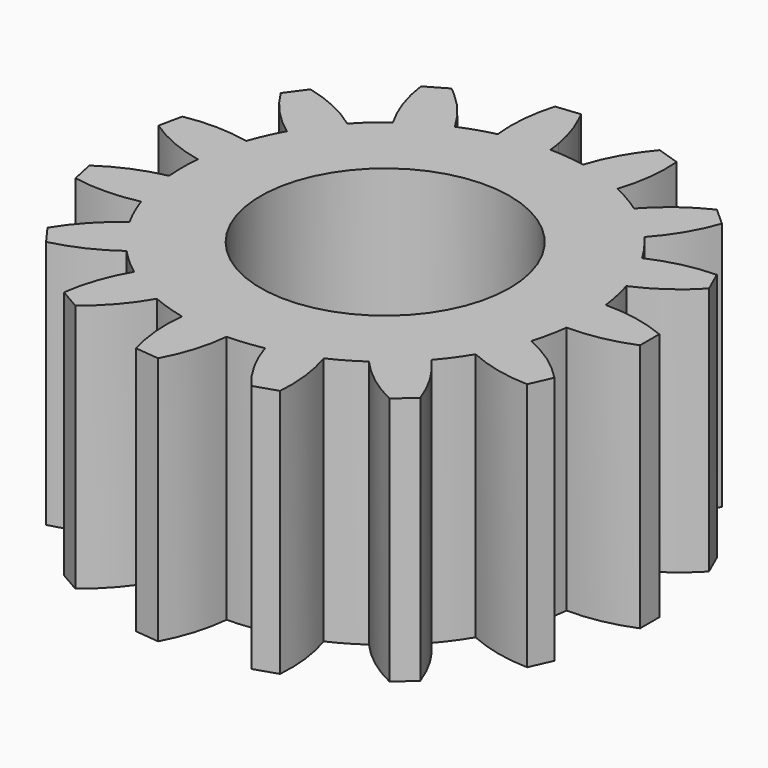
from build123d import *

# Parameters (mm, degrees)
F1_R     = 2
F2_DEPTH = 4


# Not quite as in the source:
# - a feature names something its author has since deleted; it is built from what else it names


with BuildPart() as f2:
    # F1 (on Top) → F2 (new body)
    with BuildSketch(Plane.XY):
        with BuildLine():
            ThreePointArc((-0.009331824, 3.2499866026), (0.0217852654, 3.2499269841), (0.0529003577, 3.249569441))
            ThreePointArc((0.0529003577, 3.249569441), (0.0415378352, 3.3466273722), (0.0265550076, 3.4431927066))
            ThreePointArc((0.0265550076, 3.4431927066), (0.0136878461, 3.345646772), (-0.009331824, 3.2499866026))
        make_face()
        with BuildLine():
            ThreePointArc((-0.7273678349, 3.1675599494), (-0.3706482634, 3.2287954201), (-0.009331824, 3.2499866026))
            ThreePointArc((-0.009331824, 3.2499866026), (0.0136878461, 3.345646772), (0.0265550076, 3.4431927066))
            ThreePointArc((0.0265550076, 3.4431927066), (-0.0579521884, 3.7877136915), (-0.1883330995, 4.1176182129))
            ThreePointArc((-0.1883330995, 4.1176182129), (-0.2452042442, 4.1798359688), (-0.3074340323, 4.2366939473))
            Line((-0.3074340323, 4.2366939473), (-0.6356215278, 4.2022000516))
            ThreePointArc((-0.6356215278, 4.2022000516), (-0.733410077, 3.6894835779), (-0.7273678349, 3.1675599494))
        make_face()
        with BuildLine():
            ThreePointArc((-0.3074340323, 4.2366939473), (-0.2452042442, 4.1798359688), (-0.1883330995, 4.1176182129))
            ThreePointArc((-0.1883330995, 4.1176182129), (-0.219306435, 4.1804982316), (-0.2519548455, 4.2425250448))
            Line((-0.2519548455, 4.2425250448), (-0.3074340323, 4.2366939473))
        make_face()
        with BuildLine():
            ThreePointArc((3.2262383665, -0.392283064), (3.2440541527, -0.1965010289), (3.25, 0))
            ThreePointArc((3.25, 0), (3.2440541527, 0.1965010289), (3.2262383665, 0.392283064))
            ThreePointArc((3.2262383665, 0.392283064), (3.1789797024, 0.6757129952), (3.1068713016, 0.9538609518))
            ThreePointArc((3.1068713016, 0.9538609518), (2.9690227373, 1.32189409), (2.7877595085, 1.6705977742))
            ThreePointArc((2.7877595085, 1.6705977742), (2.6293052317, 1.91030207), (2.4502979636, 2.1350737434))
            ThreePointArc((2.4502979636, 2.1350737434), (2.1746744707, 2.4152206828), (1.8672517054, 2.6600509523))
            ThreePointArc((1.8672517054, 2.6600509523), (1.625, 2.8145825623), (1.3700458474, 2.9471128883))
            ThreePointArc((1.3700458474, 2.9471128883), (1.0043052317, 3.090933678), (0.623879119, 3.189557155))
            ThreePointArc((0.623879119, 3.189557155), (0.3397175056, 3.2321961599), (0.0529003577, 3.249569441))
            ThreePointArc((0.0529003577, 3.249569441), (0.0217852654, 3.2499269841), (-0.009331824, 3.2499866026))
            ThreePointArc((-0.009331824, 3.2499866026), (-0.673671928, 2.6091227037), (-1.565226307, 2.8482567665))
            ThreePointArc((-1.565226307, 2.8482567665), (-1.7634860259, 2.7299481747), (-1.9528462821, 2.5978628521))
            ThreePointArc((-1.9528462821, 2.5978628521), (-2.1746744707, 2.4152206828), (-2.3795034667, 2.2136989976))
            ThreePointArc((-2.3795034667, 2.2136989976), (-2.6293052317, 1.91030207), (-2.8406598662, 1.5789716669))
            ThreePointArc((-2.8406598662, 1.5789716669), (-2.9690227373, 1.32189409), (-3.0741770825, 1.0544834116))
            ThreePointArc((-3.0741770825, 1.0544834116), (-3.1789797024, 0.6757129952), (-3.2372975527, 0.287061936))
            ThreePointArc((-3.2372975527, 0.287061936), (-3.25, 0), (-3.2372975527, -0.287061936))
            ThreePointArc((-3.2372975527, -0.287061936), (-3.1789797024, -0.6757129952), (-3.0741770825, -1.0544834116))
            ThreePointArc((-3.0741770825, -1.0544834116), (-2.9690227373, -1.32189409), (-2.8406598662, -1.5789716669))
            ThreePointArc((-2.8406598662, -1.5789716669), (-2.6293052317, -1.91030207), (-2.3795034667, -2.2136989976))
            ThreePointArc((-2.3795034667, -2.2136989976), (-2.1746744707, -2.4152206828), (-1.9528462821, -2.5978628521))
            ThreePointArc((-1.9528462821, -2.5978628521), (-1.625, -2.8145825623), (-1.2733920844, -2.9901459161))
            ThreePointArc((-1.2733920844, -2.9901459161), (-1.0043052317, -3.090933678), (-0.7273678349, -3.1675599494))
            ThreePointArc((-0.7273678349, -3.1675599494), (-0.3397175056, -3.2321961599), (0.0529003577, -3.249569441))
            ThreePointArc((0.0529003577, -3.249569441), (0.3397175056, -3.2321961599), (0.623879119, -3.189557155))
            ThreePointArc((0.623879119, -3.189557155), (1.0043052317, -3.090933678), (1.3700458474, -2.9471128883))
            ThreePointArc((1.3700458474, -2.9471128883), (1.625, -2.8145825623), (1.8672517054, -2.6600509523))
            ThreePointArc((1.8672517054, -2.6600509523), (2.1746744707, -2.4152206828), (2.4502979636, -2.1350737434))
            ThreePointArc((2.4502979636, -2.1350737434), (2.6293052317, -1.91030207), (2.7877595085, -1.6705977742))
            ThreePointArc((2.7877595085, -1.6705977742), (2.9690227373, -1.32189409), (3.1068713016, -0.9538609518))
            ThreePointArc((3.1068713016, -0.9538609518), (3.1789797024, -0.6757129952), (3.2262383665, -0.392283064))
        make_face()
        Circle(F1_R, mode=Mode.SUBTRACT)
        with BuildLine():
            ThreePointArc((-1.8325056355, 3.6726799025), (-1.7998502093, 3.2277290794), (-1.565226307, 2.8482567665))
            ThreePointArc((-1.565226307, 2.8482567665), (-1.4210811819, 2.9228459204), (-1.2733920844, 2.9901459161))
            ThreePointArc((-1.2733920844, 2.9901459161), (-1.5239397604, 3.3551763863), (-1.8325056355, 3.6726799025))
        make_face()
        with BuildLine():
            ThreePointArc((-1.9528462821, 2.5978628521), (-1.7634860259, 2.7299481747), (-1.565226307, 2.8482567665))
            ThreePointArc((-1.565226307, 2.8482567665), (-1.7998502093, 3.2277290794), (-1.8325056355, 3.6726799025))
            ThreePointArc((-1.8325056355, 3.6726799025), (-1.893368674, 3.7239080781), (-1.9557625995, 3.7732602156))
            Line((-1.9557625995, 3.7732602156), (-2.289857902, 3.5803702027))
            ThreePointArc((-2.289857902, 3.5803702027), (-2.1706516096, 3.0722062109), (-1.9528462821, 2.5978628521))
        make_face()
        with BuildLine():
            ThreePointArc((-2.8406598662, 1.5789716669), (-2.6293052317, 1.91030207), (-2.3795034667, 2.2136989976))
            ThreePointArc((-2.3795034667, 2.2136989976), (-2.8284814668, 2.4798935471), (-3.3214012325, 2.651564416))
            Line((-3.3214012325, 2.651564416), (-3.5481570423, 2.3394618192))
            ThreePointArc((-3.5481570423, 2.3394618192), (-3.2325677592, 1.9237164799), (-2.8406598662, 1.5789716669))
        make_face()
        with BuildLine():
            ThreePointArc((-3.2372975527, 0.287061936), (-3.1789797024, 0.6757129952), (-3.0741770825, 1.0544834116))
            ThreePointArc((-3.0741770825, 1.0544834116), (-3.5926099725, 1.1150484286), (-4.1127394185, 1.0713890403))
            Line((-4.1127394185, 1.0713890403), (-4.1929475959, 0.6940392338))
            ThreePointArc((-4.1929475959, 0.6940392338), (-3.7355435762, 0.4425986931), (-3.2372975527, 0.287061936))
        make_face()
        with BuildLine():
            ThreePointArc((-4.1127394185, -1.0713890403), (-3.5926099725, -1.1150484286), (-3.0741770825, -1.0544834116))
            ThreePointArc((-3.0741770825, -1.0544834116), (-3.1789797024, -0.6757129952), (-3.2372975527, -0.287061936))
            ThreePointArc((-3.2372975527, -0.287061936), (-3.7355435762, -0.4425986931), (-4.1929475959, -0.6940392338))
            Line((-4.1929475959, -0.6940392338), (-4.1127394185, -1.0713890403))
        make_face()
        with BuildLine():
            ThreePointArc((-3.3214012325, -2.651564416), (-2.8284814668, -2.4798935471), (-2.3795034667, -2.2136989976))
            ThreePointArc((-2.3795034667, -2.2136989976), (-2.6293052317, -1.91030207), (-2.8406598662, -1.5789716669))
            ThreePointArc((-2.8406598662, -1.5789716669), (-3.2325677592, -1.9237164799), (-3.5481570423, -2.3394618192))
            Line((-3.5481570423, -2.3394618192), (-3.3214012325, -2.651564416))
        make_face()
        with BuildLine():
            ThreePointArc((-1.9557625995, -3.7732602156), (-1.5752828195, -3.4159425422), (-1.2733920844, -2.9901459161))
            ThreePointArc((-1.2733920844, -2.9901459161), (-1.625, -2.8145825623), (-1.9528462821, -2.5978628521))
            ThreePointArc((-1.9528462821, -2.5978628521), (-2.1706516096, -3.0722062109), (-2.289857902, -3.5803702027))
            Line((-2.289857902, -3.5803702027), (-1.9557625995, -3.7732602156))
        make_face()
        with BuildLine():
            ThreePointArc((-0.2519548455, -4.2425250448), (-0.0497034617, -3.7613440389), (0.0529003577, -3.249569441))
            ThreePointArc((0.0529003577, -3.249569441), (-0.3397175056, -3.2321961599), (-0.7273678349, -3.1675599494))
            ThreePointArc((-0.7273678349, -3.1675599494), (-0.733410077, -3.6894835779), (-0.6356215278, -4.2022000516))
            Line((-0.6356215278, -4.2022000516), (-0.2519548455, -4.2425250448))
        make_face()
        with BuildLine():
            ThreePointArc((1.4954181903, -3.9782187517), (1.4844700761, -3.4563749805), (1.3700458474, -2.9471128883))
            ThreePointArc((1.3700458474, -2.9471128883), (1.0043052317, -3.090933678), (0.623879119, -3.189557155))
            ThreePointArc((0.623879119, -3.189557155), (0.8306447207, -3.6688157164), (1.128519583, -4.0974313357))
            Line((1.128519583, -4.0974313357), (1.4954181903, -3.9782187517))
        make_face()
        with BuildLine():
            ThreePointArc((2.9842198355, -3.0260422954), (2.7619652518, -2.5537672878), (2.4502979636, -2.1350737434))
            ThreePointArc((2.4502979636, -2.1350737434), (2.1746744707, -2.4152206828), (1.8672517054, -2.6600509523))
            ThreePointArc((1.8672517054, -2.6600509523), (2.2510735, -3.0137762873), (2.6975294056, -3.2841795179))
            Line((2.6975294056, -3.2841795179), (2.9842198355, -3.0260422954))
        make_face()
        with BuildLine():
            ThreePointArc((3.9570227603, -1.5506356355), (3.5618915438, -1.2095900308), (3.1068713016, -0.9538609518))
            ThreePointArc((3.1068713016, -0.9538609518), (2.9690227373, -1.32189409), (2.7877595085, -1.6705977742))
            ThreePointArc((2.7877595085, -1.6705977742), (3.2822712209, -1.8376275589), (3.8001118877, -1.9030632256))
            Line((3.8001118877, -1.9030632256), (3.9570227603, -1.5506356355))
        make_face()
        with BuildLine():
            ThreePointArc((3.2262383665, 0.392283064), (3.2440541527, 0.1965010289), (3.25, 0))
            ThreePointArc((3.25, 0), (3.2440541527, -0.1965010289), (3.2262383665, -0.392283064))
            ThreePointArc((3.2262383665, -0.392283064), (3.7459344291, -0.3437363313), (4.2456205015, -0.1928900128))
            Line((4.2456205015, -0.1928900128), (4.2456205015, 0.1928900128))
            ThreePointArc((4.2456205015, 0.1928900128), (3.7459344291, 0.3437363313), (3.2262383665, 0.392283064))
        make_face()
        with BuildLine():
            ThreePointArc((2.7877595085, 1.6705977742), (2.9690227373, 1.32189409), (3.1068713016, 0.9538609518))
            ThreePointArc((3.1068713016, 0.9538609518), (3.5618915438, 1.2095900308), (3.9570227603, 1.5506356355))
            Line((3.9570227603, 1.5506356355), (3.8001118877, 1.9030632256))
            ThreePointArc((3.8001118877, 1.9030632256), (3.2822712209, 1.8376275589), (2.7877595085, 1.6705977742))
        make_face()
        with BuildLine():
            ThreePointArc((1.8672517054, 2.6600509523), (2.1746744707, 2.4152206828), (2.4502979636, 2.1350737434))
            ThreePointArc((2.4502979636, 2.1350737434), (2.7619652518, 2.5537672878), (2.9842198355, 3.0260422954))
            Line((2.9842198355, 3.0260422954), (2.6975294056, 3.2841795179))
            ThreePointArc((2.6975294056, 3.2841795179), (2.2510735, 3.0137762873), (1.8672517054, 2.6600509523))
        make_face()
        with BuildLine():
            ThreePointArc((0.623879119, 3.189557155), (1.0043052317, 3.090933678), (1.3700458474, 2.9471128883))
            ThreePointArc((1.3700458474, 2.9471128883), (1.4844700761, 3.4563749805), (1.4954181903, 3.9782187517))
            Line((1.4954181903, 3.9782187517), (1.128519583, 4.0974313357))
            ThreePointArc((1.128519583, 4.0974313357), (0.8306447207, 3.6688157164), (0.623879119, 3.189557155))
        make_face()
        with BuildLine():
            ThreePointArc((-1.565226307, 2.8482567665), (-0.673671928, 2.6091227037), (-0.009331824, 3.2499866026))
            ThreePointArc((-0.009331824, 3.2499866026), (-0.3706482634, 3.2287954201), (-0.7273678349, 3.1675599494))
            ThreePointArc((-0.7273678349, 3.1675599494), (-1.0043052317, 3.090933678), (-1.2733920844, 2.9901459161))
            ThreePointArc((-1.2733920844, 2.9901459161), (-1.4210811819, 2.9228459204), (-1.565226307, 2.8482567665))
        make_face()
    extrude(amount=F2_DEPTH)


solid = f2.part
